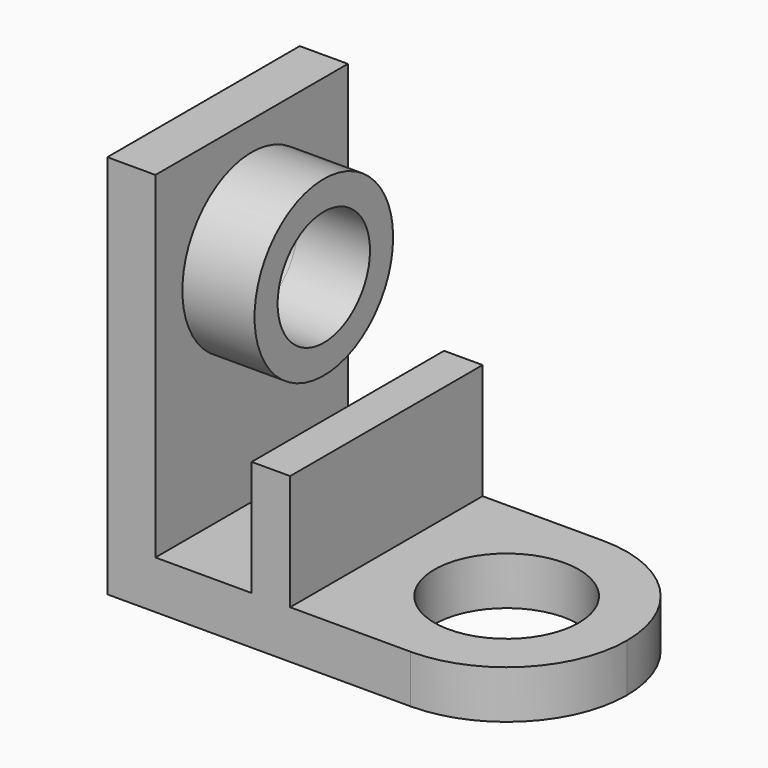
from build123d import *

# Parameters (mm, degrees)
F1_DEPTH = 50
F2_R     = 24.99999
F3_R     = 15
F4_DEPTH = 10
F5_R     = 18
F5_R_2   = 12
F6_DEPTH = 15
F7_DEPTH = 10


# Not quite as in the source:
# - a fillet or chamfer is up to 0.001 mm smaller than in the source, because OpenCascade refuses the exact size


with BuildPart() as f1:
    # F0 (on Front) → F1 (new body)
    with BuildSketch(Plane.XZ):
        Polygon((0, 80), (0, 0), (88, 0), (88, 10), (38, 10), (38, 34), (30, 34), (30, 10), (10, 10), (10, 80), align=None)
    extrude(amount=F1_DEPTH)

    # F2 (radius 25 in the source; OpenCascade refuses exactly that, so slightly less here)
    f2_edges = [f1.edges().sort_by_distance(p)[0] for p in [
        (88, -50, 5),
        (88, 0, 5),
    ]]
    fillet(f2_edges, radius=F2_R)

    # F3 (on face) → F4 (cut, through all)
    with BuildSketch(Plane.XY.offset(10)):
        with Locations((63, -25)):
            Circle(F3_R)
    extrude(amount=-F4_DEPTH, mode=Mode.SUBTRACT)

    # F5 (on face) → F6 (join)
    with BuildSketch(Plane.YZ.offset(10)):
        with Locations((-25, 56)):
            Circle(F5_R)
        with Locations((-25, 56)):
            Circle(F5_R_2, mode=Mode.SUBTRACT)
    extrude(amount=F6_DEPTH)

    # F7 (cut, through all): a face of the model
    f7_faces = [f1.faces().sort_by_distance(p)[0] for p in [
        (10, -25, 56),
    ]]
    extrude(f7_faces, amount=-F7_DEPTH, mode=Mode.SUBTRACT)


solid = f1.part
